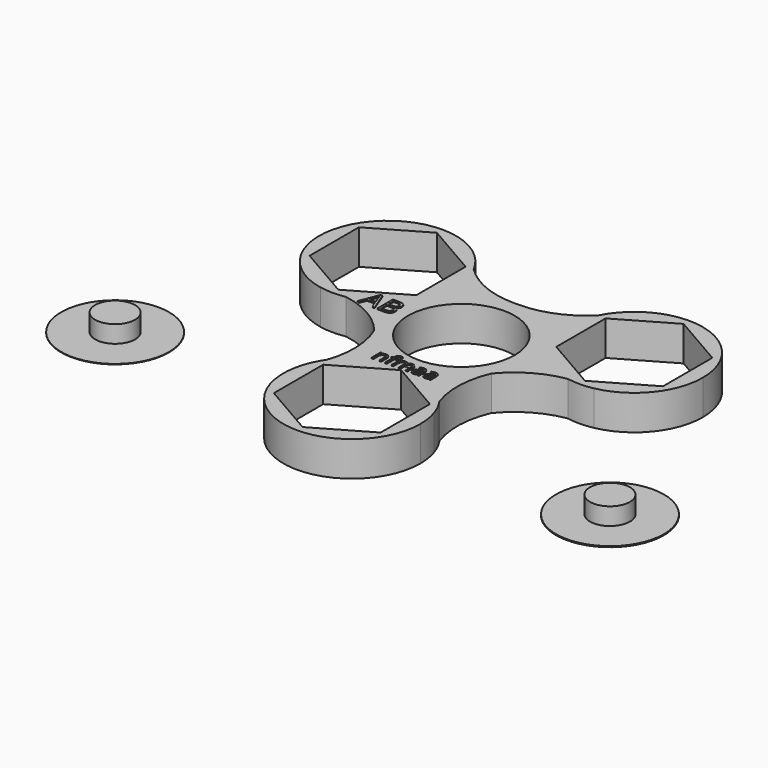
from build123d import *

# Parameters (mm, degrees)
F0_R           = 10.7304815216
F1_DEPTH       = 7
F2_TEXT_SIZE   = 4.1746185161
F2_TEXT_SIZE_2 = 5.4782359964
F4_DEPTH       = 7.15
F3_R           = 10.8372934451
F3_R_2         = 4.0101369685
F5_DEPTH       = 0.1
F6_DEPTH       = 3.58
F7_DEPTH       = 0.2
F8_DEPTH       = 3.69


# Not quite as in the source:
# - Text() gives the source's letters only with a copy of the font that has no kerning and outlines rounded to 1/6400 em; it was checked with that copy


with BuildPart() as f1:
    # F0 (on Top) → F1 (new body)
    with BuildSketch(Plane.XY):
        with BuildLine():
            ThreePointArc((0.9233610876, -13.7511929497), (7.1517444138, -11.7813604935), (11.7734430895, -7.1647708307))
            ThreePointArc((11.7734430895, -7.1647708307), (13.2704816491, -3.7205134108), (13.7821588744, 0))
            ThreePointArc((13.7821588744, 0), (9.8895943929, 9.5991575663), (0.4106940954, 13.7760383855))
            ThreePointArc((0.4106940954, 13.7760383855), (0.205328652, 13.7778642495), (0, 13.7821588744))
            ThreePointArc((0, 13.7821588744), (-0.205328652, 13.7778642495), (-0.4106940954, 13.7760383855))
            ThreePointArc((-0.4106940954, 13.7760383855), (-12.1137389931, 6.573068602), (-11.7734430895, -7.1647708307))
            ThreePointArc((-11.7734430895, -7.1647708307), (-7.1517444138, -11.7813604935), (-0.9233610876, -13.7511929497))
            ThreePointArc((-0.9233610876, -13.7511929497), (0, -13.7202270251), (0.9233610876, -13.7511929497))
        make_face()
        Circle(F0_R, mode=Mode.SUBTRACT)
        with BuildLine():
            ThreePointArc((11.339891833, -19.6694581931), (10.3706023054, -13.3759923291), (11.7734430895, -7.1647708307))
            ThreePointArc((11.7734430895, -7.1647708307), (7.1517444138, -11.7813604935), (0.9233610876, -13.7511929497))
            ThreePointArc((0.9233610876, -13.7511929497), (6.8083264406, -15.5192897087), (11.339891833, -19.6694581931))
        make_face()
        with BuildLine():
            ThreePointArc((13.7821588744, 0), (13.2704816491, -3.7205134108), (11.7734430895, -7.1647708307))
            ThreePointArc((11.7734430895, -7.1647708307), (16.4877063172, -3.152839634), (22.3221878913, -1.0843390979))
            ThreePointArc((22.3221878913, -1.0843390979), (12.4310485225, 6.3889110276), (12.5452102886, 18.7853247244))
            ThreePointArc((12.5452102886, 18.7853247244), (6.9783486661, 15.0685190418), (0.4106940954, 13.7760383855))
            ThreePointArc((0.4106940954, 13.7760383855), (9.8895943929, 9.5991575663), (13.7821588744, 0))
        make_face()
        with BuildLine():
            ThreePointArc((11.339891833, -19.6694581931), (6.8083264406, -15.5192897087), (0.9233610876, -13.7511929497))
            ThreePointArc((0.9233610876, -13.7511929497), (0, -13.7821588744), (-0.9233610876, -13.7511929497))
            ThreePointArc((-0.9233610876, -13.7511929497), (-6.8083264406, -15.5192897087), (-11.339891833, -19.6694581931))
            ThreePointArc((-11.339891833, -19.6694581931), (-12.1222682503, -21.5239245291), (-13.1173322992, -23.2734975594))
            ThreePointArc((-13.1173322992, -23.2734975594), (-2.1404141519, -41.11732367), (13.7821588744, -27.5023858994))
            ThreePointArc((13.7821588744, -27.5023858994), (13.6149377706, -25.3619717475), (13.1173322992, -23.2734975594))
            ThreePointArc((13.1173322992, -23.2734975594), (12.1222682503, -21.5239245291), (11.339891833, -19.6694581931))
        make_face()
        Polygon((0, -15.1118931094), (10.7304815216, -21.3071395044), (10.7304815216, -33.6976322945), (0, -39.8928786895), (-10.7304815216, -33.6976322945), (-10.7304815216, -21.3071395044), align=None, mode=Mode.SUBTRACT)
        with BuildLine():
            ThreePointArc((27.4694220966, -1.0468650982), (24.8943854484, -0.8706206898), (22.3221878913, -1.0843390979))
            ThreePointArc((22.3221878913, -1.0843390979), (24.8975699948, -1.3080334584), (27.4694220966, -1.0468650982))
        make_face()
        with BuildLine():
            ThreePointArc((12.5452102886, 18.7853247244), (12.4310485225, 6.3889110276), (22.3221878913, -1.0843390979))
            ThreePointArc((22.3221878913, -1.0843390979), (24.8943854484, -0.8706206898), (27.4694220966, -1.0468650982))
            ThreePointArc((27.4694220966, -1.0468650982), (35.4456233189, 3.7239211425), (38.579391696, 12.4737601727))
            ThreePointArc((38.579391696, 12.4737601727), (30.2798185579, 25.1184885954), (15.3770533192, 22.533984891))
            ThreePointArc((15.3770533192, 22.533984891), (14.090614185, 20.5618401853), (12.5452102886, 18.7853247244))
        make_face()
        Polygon((24.7972328216, 0.0832673827), (14.0667513, 6.2785137777), (14.0667513, 18.6690065678), (24.7972328216, 24.8642529628), (35.5277143432, 18.6690065678), (35.5277143432, 6.2785137777), align=None, mode=Mode.SUBTRACT)
        with BuildLine():
            ThreePointArc((13.1173322992, -23.2734975594), (12.3606726355, -21.4063482325), (11.339891833, -19.6694581931))
            ThreePointArc((11.339891833, -19.6694581931), (12.1222682503, -21.5239245291), (13.1173322992, -23.2734975594))
        make_face()
        with BuildLine():
            ThreePointArc((0, 13.7821588744), (0.205328652, 13.7778642495), (0.4106940954, 13.7760383855))
            ThreePointArc((0.4106940954, 13.7760383855), (0.2053698495, 13.7806286672), (0, 13.7821588744))
        make_face()
        with BuildLine():
            ThreePointArc((-11.339891833, -19.6694581931), (-6.8083264406, -15.5192897087), (-0.9233610876, -13.7511929497))
            ThreePointArc((-0.9233610876, -13.7511929497), (-7.1517444138, -11.7813604935), (-11.7734430895, -7.1647708307))
            ThreePointArc((-11.7734430895, -7.1647708307), (-10.3706023054, -13.3759923291), (-11.339891833, -19.6694581931))
        make_face()
        with BuildLine():
            ThreePointArc((15.3770533192, 22.533984891), (13.8002242044, 20.7812089214), (12.5452102886, 18.7853247244))
            ThreePointArc((12.5452102886, 18.7853247244), (14.090614185, 20.5618401853), (15.3770533192, 22.533984891))
        make_face()
        with BuildLine():
            ThreePointArc((-0.4106940954, 13.7760383855), (-0.205328652, 13.7778642495), (0, 13.7821588744))
            ThreePointArc((0, 13.7821588744), (-0.2053698495, 13.7806286672), (-0.4106940954, 13.7760383855))
        make_face()
        with BuildLine():
            ThreePointArc((-22.3221878913, -1.0843390979), (-16.4877063172, -3.152839634), (-11.7734430895, -7.1647708307))
            ThreePointArc((-11.7734430895, -7.1647708307), (-12.1137389931, 6.573068602), (-0.4106940954, 13.7760383855))
            ThreePointArc((-0.4106940954, 13.7760383855), (-6.9783486661, 15.0685190418), (-12.5452102886, 18.7853247244))
            ThreePointArc((-12.5452102886, 18.7853247244), (-11.4030694599, 15.7209575918), (-11.0150739472, 12.4737601727))
            ThreePointArc((-11.0150739472, 12.4737601727), (-14.2128252877, 3.6466303791), (-22.3221878913, -1.0843390979))
        make_face()
        with BuildLine():
            ThreePointArc((-13.1173322992, -23.2734975594), (-12.1222682503, -21.5239245291), (-11.339891833, -19.6694581931))
            ThreePointArc((-11.339891833, -19.6694581931), (-12.3606726355, -21.4063482325), (-13.1173322992, -23.2734975594))
        make_face()
        with BuildLine():
            ThreePointArc((-27.4694220966, -1.0468650982), (-24.8943854484, -0.8706206898), (-22.3221878913, -1.0843390979))
            ThreePointArc((-22.3221878913, -1.0843390979), (-14.2128252877, 3.6466303791), (-11.0150739472, 12.4737601727))
            ThreePointArc((-11.0150739472, 12.4737601727), (-11.4030694599, 15.7209575918), (-12.5452102886, 18.7853247244))
            ThreePointArc((-12.5452102886, 18.7853247244), (-14.090614185, 20.5618401853), (-15.3770533192, 22.533984891))
            ThreePointArc((-15.3770533192, 22.533984891), (-37.0609176096, 18.7626343691), (-27.4694220966, -1.0468650982))
        make_face()
        Polygon((-24.7972328216, 24.8642529628), (-14.0667513, 18.6690065678), (-14.0667513, 6.2785137777), (-24.7972328216, 0.0832673827), (-35.5277143432, 6.2785137777), (-35.5277143432, 18.6690065678), align=None, mode=Mode.SUBTRACT)
        with BuildLine():
            ThreePointArc((-27.4694220966, -1.0468650982), (-24.8975699948, -1.3080334584), (-22.3221878913, -1.0843390979))
            ThreePointArc((-22.3221878913, -1.0843390979), (-24.8943854484, -0.8706206898), (-27.4694220966, -1.0468650982))
        make_face()
        with BuildLine():
            ThreePointArc((-15.3770533192, 22.533984891), (-14.090614185, 20.5618401853), (-12.5452102886, 18.7853247244))
            ThreePointArc((-12.5452102886, 18.7853247244), (-13.8002242044, 20.7812089214), (-15.3770533192, 22.533984891))
        make_face()
    extrude(amount=F1_DEPTH)

    # F2 (on Top) → F4 (join)
    with BuildSketch(Plane.XY):
        with Locations((-6.4623090439, -14.8783409968)):
            Text('nfmaa', F2_TEXT_SIZE, font='Open Sans', text_align=(TextAlign.LEFT, TextAlign.BOTTOM))
        with Locations((-19.8489287868, -1.2974289712)):
            Text('AB', F2_TEXT_SIZE_2, font='Open Sans', text_align=(TextAlign.LEFT, TextAlign.BOTTOM))
    extrude(amount=F4_DEPTH)


with BuildPart() as f5:
    # F3 (on Top) → F5 (new body)
    with BuildSketch(Plane.XY):
        with Locations((-51.4427497983, -22.6999912411)):
            Circle(F3_R)
        with Locations((-51.4427497983, -22.6999912411)):
            Circle(F3_R_2, mode=Mode.SUBTRACT)
    extrude(amount=F5_DEPTH)

    # F3 (on Top) → F6 (join)
    with BuildSketch(Plane.XY):
        with Locations((-51.4427497983, -22.6999912411)):
            Circle(F3_R_2)
    extrude(amount=F6_DEPTH)


with BuildPart() as f7:
    # F3 (on Top) → F7 (new body)
    with BuildSketch(Plane.XY):
        with Locations((48.0467528105, -22.6999912411)):
            Circle(F3_R)
        with Locations((48.0467528105, -22.6999912411)):
            Circle(F3_R_2, mode=Mode.SUBTRACT)
    extrude(amount=F7_DEPTH)

    # F3 (on Top) → F8 (join)
    with BuildSketch(Plane.XY):
        with Locations((48.0467528105, -22.6999912411)):
            Circle(F3_R_2)
    extrude(amount=F8_DEPTH)


solid = Compound([f1.part, f5.part, f7.part])
